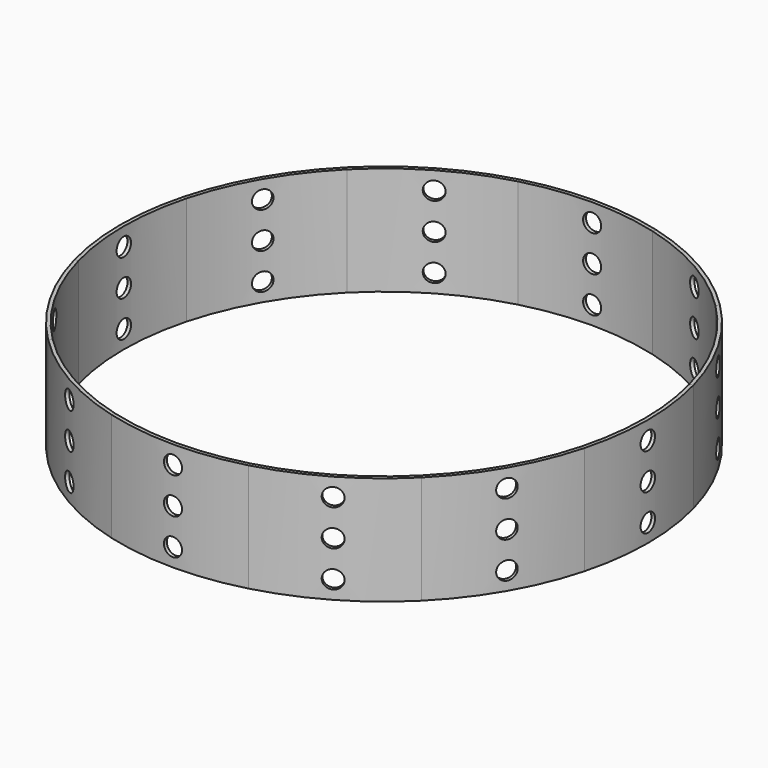
from build123d import *
from build123d import SkipClean  # not in build123d's __all__

# Parameters (mm, degrees)
F0_W          = 1
F0_H          = 30
F1_ANGLE_BACK = 15
F1_ANGLE      = 30
F2_R          = 2.5
F3_DEPTH      = 75
F4_COUNT      = 12


with BuildPart() as f1:
    # F0 (on Front) → F1 (revolve)
    with BuildSketch(Plane.XZ, mode=Mode.PRIVATE) as f1_sk:
        with Locations((-72.5, 15)):
            Rectangle(F0_W, F0_H)
    revolve(f1_sk.sketch.rotate(Axis((0, 0, 16.7500004172), (0, 0, 1)), -F1_ANGLE_BACK), axis=Axis((0, 0, 16.7500004172), (0, 0, 1)), revolution_arc=F1_ANGLE)

    # F2 (on Right) → F3 (cut)
    with BuildSketch(Plane.YZ):
        with Locations((0, 5)):
            Circle(F2_R)
        with Locations((0, 15)):
            Circle(F2_R)
        with Locations((0, 25)):
            Circle(F2_R)
    extrude(amount=-F3_DEPTH, mode=Mode.SUBTRACT)

    # F4: F1 ×12 about axis
    f4_axis = Axis((0, 0, 16.7500004172), (0, 0, 1))


with BuildPart() as f1_1:
    add(f1.part, clean=False)
    with SkipClean():  # cleaning this boolean's faces spoils the solid; the shape is the same uncleaned
        for i in range(1, F4_COUNT):
            add(f1.part.rotate(f4_axis, i * 360 / F4_COUNT), clean=False)


solid = f1_1.part
